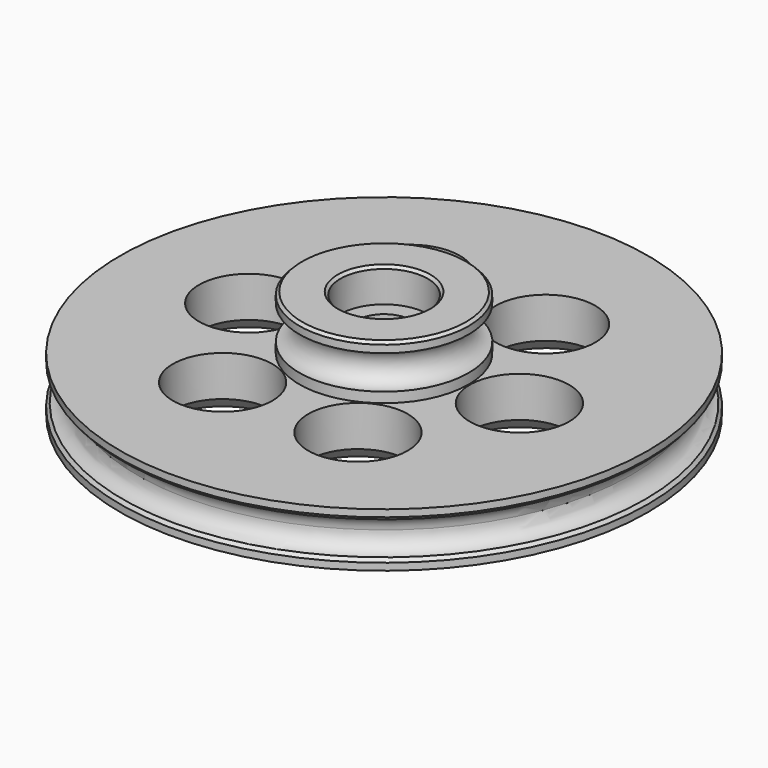
from build123d import *

# Parameters (mm, degrees)
F0_R        = 39
F0_R_2      = 2.325
F1_DEPTH    = 4
F2_R        = 2.5
F4_T2_ANGLE = 270
F4_T4_ANGLE = 90
F4_T6_ANGLE = 90
F4_T8_ANGLE = 270
F5_R        = 7.35
F6_DEPTH    = 25
F7_SIZE     = 2
F8_R        = 12.5
F9_DEPTH    = 8
F12_R       = 6.45
F13_DEPTH   = 5
F14_R       = 6.45
F15_DEPTH   = 5
F16_SIZE    = 0.4
F17_R       = 4
F18_DEPTH   = 11.001


# Not quite as in the source:
# - a fillet or chamfer that OpenCascade refuses, or shapes differently, is made with other operations: its cross-section is extruded or revolved along the edge and cut away or added
# - a feature names something its author has since deleted; it is built from what else it names


with BuildPart() as f1:
    # F0 (on Top) → F1 (new body, symmetric)
    with BuildSketch(Plane.XY):
        Circle(F0_R)
        Circle(F0_R_2, mode=Mode.SUBTRACT)
    extrude(amount=F1_DEPTH, both=True)

    # F2 (on Right) → F3 (revolve, cut)
    with BuildSketch(Plane.YZ):
        with Locations((-39, 0)):
            Circle(F2_R)
    revolve(axis=Axis((0, 0, 0), (0, 0, -1)), mode=Mode.SUBTRACT)

    # F4: chamfer of 0.5 on 4 edges, made by hand

    # F4_s1 → F4_t2 (revolve, cut)
    with BuildSketch(Plane.YZ):
        with BuildLine():
            Line((-39, -2.9580398915), (-38.5833333333, -2.465033243))
            ThreePointArc((-38.5833333333, -2.465033243), (-38.7838440297, -2.4906377891), (-39, -2.5))
            Line((-39, -2.5), (-39, -2.9580398915))
        make_face()
    revolve(axis=Axis((0, 0, -2.5), (0, 0, -1)), revolution_arc=F4_T2_ANGLE, mode=Mode.SUBTRACT)

    # F4_s3 → F4_t4 (revolve, cut)
    with BuildSketch(Plane.XZ):
        with BuildLine():
            Line((39, -2.9580398915), (38.5833333333, -2.465033243))
            ThreePointArc((38.5833333333, -2.465033243), (38.7838440297, -2.4906377891), (39, -2.5))
            Line((39, -2.5), (39, -2.9580398915))
        make_face()
    revolve(axis=Axis((0, 0, -2.5), (0, 0, -1)), revolution_arc=F4_T4_ANGLE, mode=Mode.SUBTRACT)

    # F4_s5 → F4_t6 (revolve, cut)
    with BuildSketch(Plane.XZ):
        with BuildLine():
            Line((38.5833333333, 2.465033243), (39, 2.9580398915))
            Line((39, 2.9580398915), (39, 2.5))
            ThreePointArc((39, 2.5), (38.7838440297, 2.4906377891), (38.5833333333, 2.465033243))
        make_face()
    revolve(axis=Axis((0, 0, 2.5), (0, 0, -1)), revolution_arc=F4_T6_ANGLE, mode=Mode.SUBTRACT)

    # F4_s7 → F4_t8 (revolve, cut)
    with BuildSketch(Plane.YZ):
        with BuildLine():
            Line((-38.5833333333, 2.465033243), (-39, 2.9580398915))
            Line((-39, 2.9580398915), (-39, 2.5))
            ThreePointArc((-39, 2.5), (-38.7838440297, 2.4906377891), (-38.5833333333, 2.465033243))
        make_face()
    revolve(axis=Axis((0, 0, 2.5), (0, 0, -1)), revolution_arc=F4_T8_ANGLE, mode=Mode.SUBTRACT)

    # F5 (on face) → F6 (cut)
    with BuildSketch(Plane.XY.offset(4)):
        with Locations((20, 0)):
            Circle(F5_R)
        with Locations((10, -17.3205080757)):
            Circle(F5_R)
        with Locations((-10, -17.3205080757)):
            Circle(F5_R)
        with Locations((-20, 0)):
            Circle(F5_R)
        with Locations((-10, 17.3205080757)):
            Circle(F5_R)
        with Locations((10, 17.3205080757)):
            Circle(F5_R)
    extrude(amount=-F6_DEPTH, mode=Mode.SUBTRACT)

    # F7
    f7_edges = [f1.edges().sort_by_distance(p)[0] for p in [
        (-27.35, 0, -4),
        (-17.35, -17.320508, -4),
        (2.65, -17.320508, -4),
        (12.65, 0, -4),
        (2.65, 17.320508, -4),
        (-17.35, 17.320508, -4),
    ]]
    chamfer(f7_edges, length=F7_SIZE)

    # F8 (on face) → F9 (join)
    with BuildSketch(Plane.XY.offset(4)):
        Circle(F8_R)
    extrude(amount=F9_DEPTH)

    # F10 (on Right) → F11 (revolve, cut)
    with BuildSketch(Plane.YZ):
        with BuildLine():
            Line((12.5, 5.5), (12.5, 10.5))
            ThreePointArc((12.5, 10.5), (10, 8), (12.5, 5.5))
        make_face()
    revolve(axis=Axis((0, 0, 4), (0, 0, -1)), mode=Mode.SUBTRACT)

    # F12 (on face) → F13 (cut)
    with BuildSketch(Plane.XY.offset(12)):
        Circle(F12_R)
    extrude(amount=-F13_DEPTH, mode=Mode.SUBTRACT)

    # F14 (on face) → F15 (cut)
    with BuildSketch(Plane(origin=(0, 0, -4), x_dir=(1, 0, 0), z_dir=(0, 0, -1))):
        Circle(F14_R)
    extrude(amount=-F15_DEPTH, mode=Mode.SUBTRACT)

    # F16
    f16_edges = [f1.edges().sort_by_distance(p)[0] for p in [
        (-12.5, 0, 12),
        (-6.45, 0, 12),
        (-6.45, 0, -4),
    ]]
    chamfer(f16_edges, length=F16_SIZE)

    # F17 (on face) → F18 (cut, through all)
    with BuildSketch(Plane.XY.offset(7)):
        Circle(F17_R)
    extrude(amount=-F18_DEPTH, mode=Mode.SUBTRACT)


solid = f1.part
